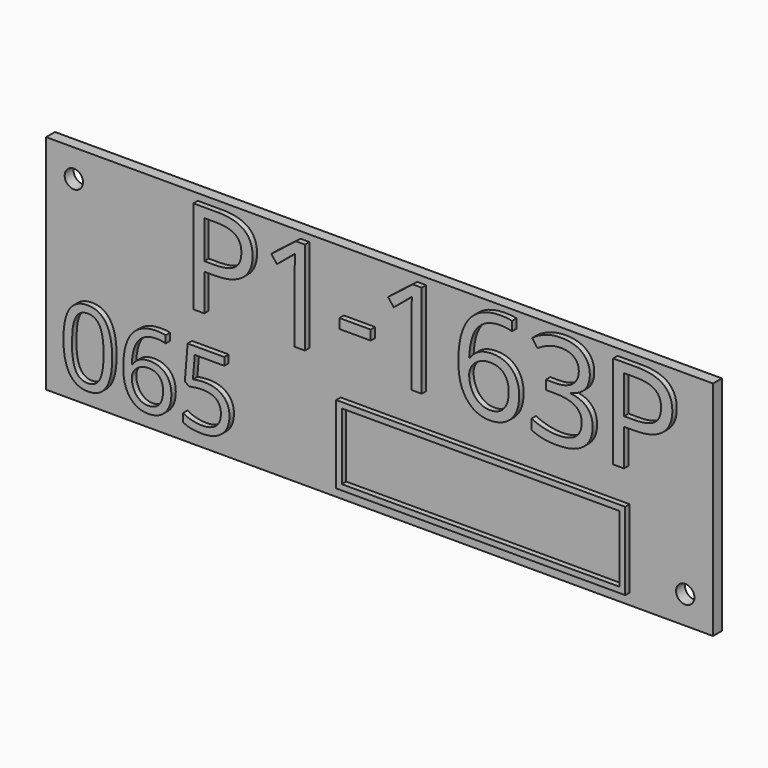
from build123d import *

# Parameters (mm, degrees)
F0_W         = 120
F0_H         = 40
F1_DEPTH     = 2
F3_D         = 3.3
F4_TEXT_SIZE = 23.5217249265
F5_DEPTH     = 1
F6_TEXT_SIZE = 18.5776487663
F7_DEPTH     = 1
F8_W         = 52
F8_H         = 14
F8_W_2       = 49.99999962
F8_H_2       = 11.99999962
F9_DEPTH     = 1


# Not quite as in the source:
# - Text() gives the source's letters only with a copy of the font that has no kerning and outlines rounded to 1/6400 em; it was checked with that copy


with BuildPart() as f1:
    # F0 (on Front) → F1 (new body)
    with BuildSketch(Plane.XZ):
        Rectangle(F0_W, F0_H)
    extrude(amount=F1_DEPTH)

    # F3 (through all)
    with Locations(Plane.XZ.offset(2)):
        with Locations((-55, 15), (55, -15)):
            Hole(F3_D / 2)

    # F4 (on face) → F5 (join)
    with BuildSketch(Plane.XZ.offset(2)):
        with Locations((-35, 2)):
            Text('P1-163P', F4_TEXT_SIZE, font='Open Sans', text_align=(TextAlign.LEFT, TextAlign.BOTTOM))
    extrude(amount=F5_DEPTH)

    # F6 (on face) → F7 (join)
    with BuildSketch(Plane.XZ.offset(2)):
        with Locations((-57, -17)):
            Text('065', F6_TEXT_SIZE, font='Open Sans', text_align=(TextAlign.LEFT, TextAlign.BOTTOM))
    extrude(amount=F7_DEPTH)

    # F8 (on face) → F9 (join)
    with BuildSketch(Plane.XZ.offset(2)):
        with Locations((19, -11)):
            Rectangle(F8_W, F8_H)
        with Locations((19, -11)):
            Rectangle(F8_W_2, F8_H_2, mode=Mode.SUBTRACT)
    extrude(amount=F9_DEPTH)


solid = f1.part
